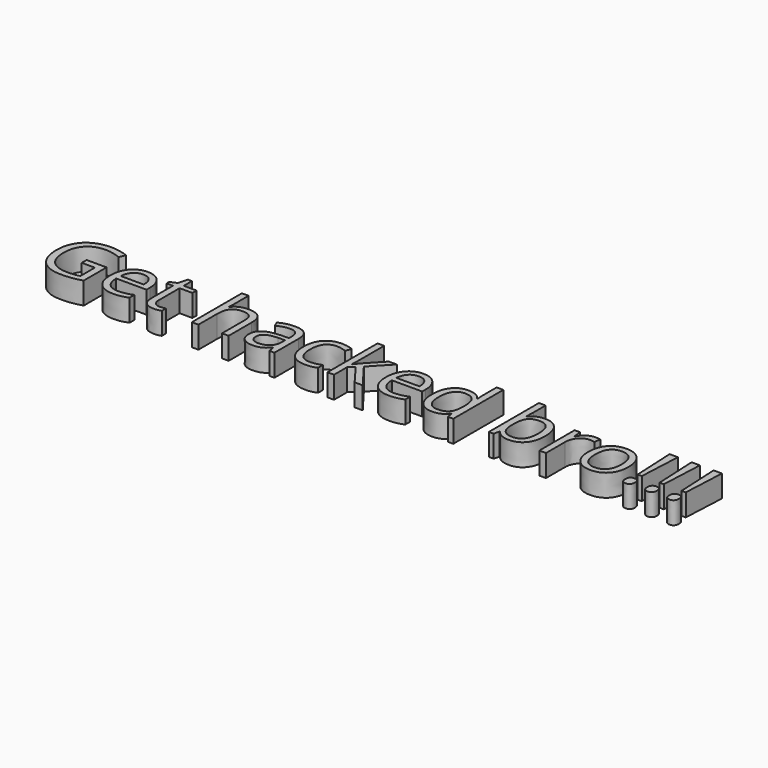
from build123d import *

# Parameters (mm, degrees)
F0_TEXT_SIZE = 94.8477795141
F1_DEPTH     = 25.4


# Not quite as in the source:
# - Text() gives the source's letters only with a copy of the font that has no kerning and outlines rounded to 1/6400 em; it was checked with that copy


with BuildPart() as f1:
    # F0 (on Top) → F1 (new body)
    with BuildSketch(Plane.XY):
        with Locations((-116.6891679168, -31.2311388552)):
            Text('Get hacked bro!!!', F0_TEXT_SIZE, font='Open Sans', text_align=(TextAlign.LEFT, TextAlign.BOTTOM))
    extrude(amount=F1_DEPTH)


solid = f1.part
